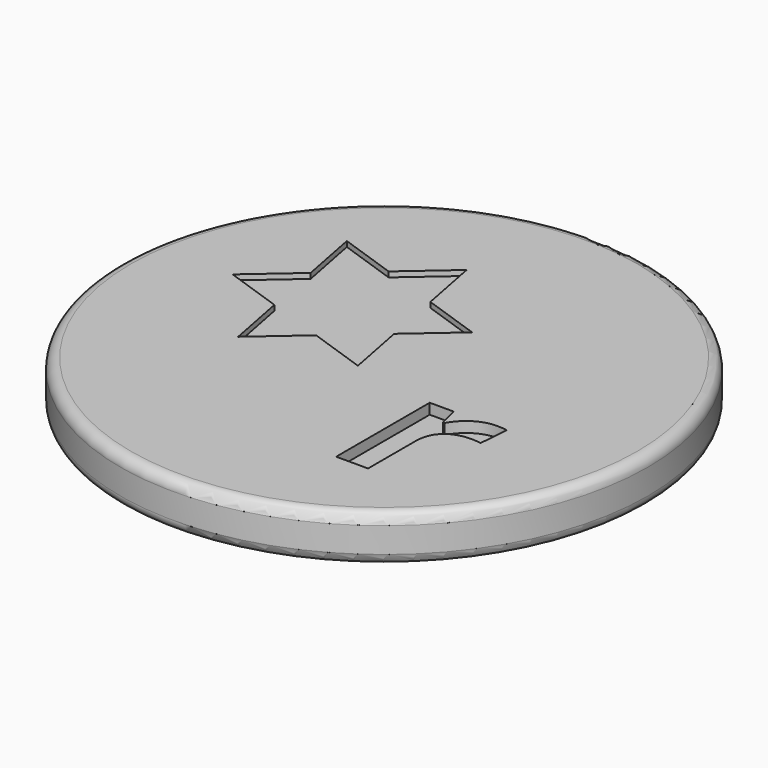
from build123d import *

# Parameters (mm, degrees)
F0_R         = 12.5
F1_DEPTH     = 2.2
F2_R         = 0.5
F3_R         = 0.5
F5_DEPTH     = 0.25
F6_TEXT_SIZE = 10.1428319211
F7_DEPTH     = 0.5


# Not quite as in the source:
# - Text() gives the source's letters only with a copy of the font that has no kerning and outlines rounded to 1/6400 em; it was checked with that copy


with BuildPart() as f1:
    # F0 (on Top) → F1 (new body)
    with BuildSketch(Plane.XY):
        Circle(F0_R)
    extrude(amount=F1_DEPTH)

    # F2
    f2_edges = [f1.edges().sort_by_distance(p)[0] for p in [
        (-12.5, 0, 2.2),
    ]]
    fillet(f2_edges, radius=F2_R)

    # F3
    f3_edges = [f1.edges().sort_by_distance(p)[0] for p in [
        (-12.5, 0, 0),
    ]]
    fillet(f3_edges, radius=F3_R)

    # F4 (on face) → F5 (cut, symmetric)
    with BuildSketch(Plane.XY.offset(2.2)):
        Polygon((-3.0784096558, -0.1736559051), (-0.3487835335, -1.1130570794), (-0.9000513134, 1.7205690724), align=None)
        Polygon((-5.2567679981, -2.0678808827), (-3.0784096558, -0.1736559051), (-5.808035778, 0.7657452691), align=None)
        Polygon((-5.808035778, 0.7657452691), (-3.0784096558, -0.1736559051), (-0.9000513134, 1.7205690724), (-1.4513190933, 4.5541952242), (-4.1809452155, 5.4935963985), (-6.3593035579, 3.5993714209), align=None)
        Polygon((-1.4513190933, 4.5541952242), (-0.9000513134, 1.7205690724), (1.2783070289, 3.61479405), align=None)
        Polygon((-8.5376619002, 1.7051464433), (-5.808035778, 0.7657452691), (-6.3593035579, 3.5993714209), align=None)
        Polygon((-4.1809452155, 5.4935963985), (-1.4513190933, 4.5541952242), (-2.0025868732, 7.387821376), align=None)
        Polygon((-6.9105713378, 6.4329975727), (-6.3593035579, 3.5993714209), (-4.1809452155, 5.4935963985), align=None)
    extrude(amount=F5_DEPTH, both=True, mode=Mode.SUBTRACT)

    # F6 (on face) → F7 (cut, symmetric)
    with BuildSketch(Plane.XY.offset(2.2)):
        with Locations((2.780763963, -7.3028389832)):
            Text('r', F6_TEXT_SIZE, font='Open Sans', font_style=FontStyle.BOLD, text_align=(TextAlign.LEFT, TextAlign.BOTTOM))
    extrude(amount=F7_DEPTH, both=True, mode=Mode.SUBTRACT)


solid = f1.part
